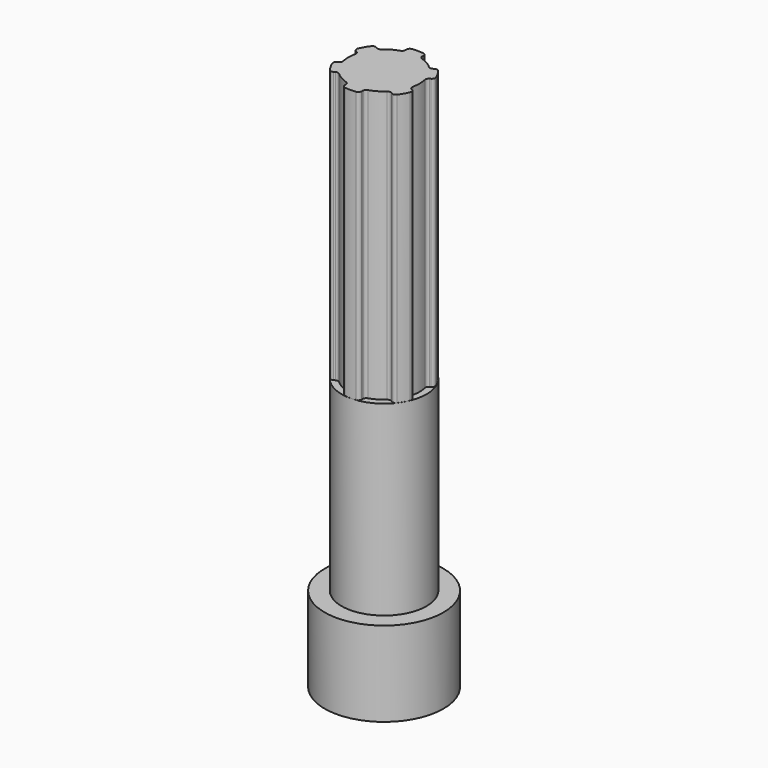
from build123d import *

# Parameters (mm, degrees)
F0_R            = 8.89
F1_DEPTH        = 12.7
F2_R            = 6.35
F3_DEPTH        = 27.94
F4_R            = 5.334
F5_DEPTH        = 40.64
F7_DEPTH        = 40.64
F7_COPIES_COUNT = 6
F8_R            = 0.508
F9_R            = 4
F10_DEPTH       = 33.02
F14_D           = 2.2606
F14_DEPTH       = 8.89
F14_START       = 0.0721476
F14_TIP         = 0.6791527577


# Not quite as in the source:
# - a pattern or mirror of a feature is missing from the dataset's text; its kind, count and spacing are read off the source's solid


with BuildPart() as f1:
    # F0 (on Top) → F1 (new body)
    with BuildSketch(Plane.XY):
        Circle(F0_R)
    extrude(amount=F1_DEPTH)

    # F2 (on face) → F3 (join)
    with BuildSketch(Plane.XY.offset(12.7)):
        Circle(F2_R)
    extrude(amount=F3_DEPTH)

    # F4 (on face) → F5 (join)
    with BuildSketch(Plane.XY.offset(40.64)):
        Circle(F4_R)
    extrude(amount=F5_DEPTH)

    # F6 (on face) → F7 (join, through all)
    with BuildSketch(Plane.XY.offset(81.28)):
        with BuildLine():
            Line((-1.27, -5.1806038258), (-1.27, -6.1957780109))
            ThreePointArc((-1.27, -6.1957780109), (0, -6.3246), (1.27, -6.1957780109))
            Line((1.27, -6.1957780109), (1.27, -5.1806038258))
            ThreePointArc((1.27, -5.1806038258), (0, -5.334), (-1.27, -5.1806038258))
        make_face()
    f7 = extrude(amount=-F7_DEPTH)

    # F7_copies: F7 ×6 about axis
    f7_copies_axis = Axis((0, 0, 0), (0, 0, 1))
    for i in range(1, F7_COPIES_COUNT):
        add(f7.rotate(f7_copies_axis, i * 360 / F7_COPIES_COUNT))

    # F8
    f8_edges = [f1.edges().sort_by_distance(p)[0] for p in [
        (1.27, -6.195778, 60.96),
        (1.27, -5.180604, 60.96),
        (-1.27, -6.195778, 60.96),
        (-1.27, -5.180604, 60.96),
        (3.851535, -3.690154, 60.96),
        (4.730701, -4.197741, 60.96),
        (6.000701, -1.998037, 60.96),
        (5.121535, -1.49045, 60.96),
        (5.121535, 1.49045, 60.96),
        (6.000701, 1.998037, 60.96),
        (4.730701, 4.197741, 60.96),
        (3.851535, 3.690154, 60.96),
        (1.27, 5.180604, 60.96),
        (1.27, 6.195778, 60.96),
        (-1.27, 6.195778, 60.96),
        (-1.27, 5.180604, 60.96),
        (-3.851535, 3.690154, 60.96),
        (-4.730701, 4.197741, 60.96),
        (-6.000701, 1.998037, 60.96),
        (-5.121535, 1.49045, 60.96),
        (-5.121535, -1.49045, 60.96),
        (-6.000701, -1.998037, 60.96),
        (-4.730701, -4.197741, 60.96),
        (-3.851535, -3.690154, 60.96),
    ]]
    fillet(f8_edges, radius=F8_R)

    # F9 (on face) → F10 (cut)
    with BuildSketch(Plane(origin=(0, 0, 0), x_dir=(1, 0, 0), z_dir=(0, 0, -1))):
        Circle(F9_R)
    extrude(amount=-F10_DEPTH, mode=Mode.SUBTRACT)

    # F14
    # its depths count from where the whole tool has entered the part; down to there all is cleared
    with Locations(Plane(origin=(-8.89, 0, 0), x_dir=(0, 1, 0), z_dir=(-1, 0, 0)).offset(-F14_START)):
        with Locations((0, -7.62)):
            Hole(F14_D / 2, depth=F14_DEPTH)
            with Locations((0, 0, -(F14_DEPTH + F14_TIP / 2))):  # 118° drill point
                Cone(0, F14_D / 2, F14_TIP, mode=Mode.SUBTRACT)


solid = f1.part
